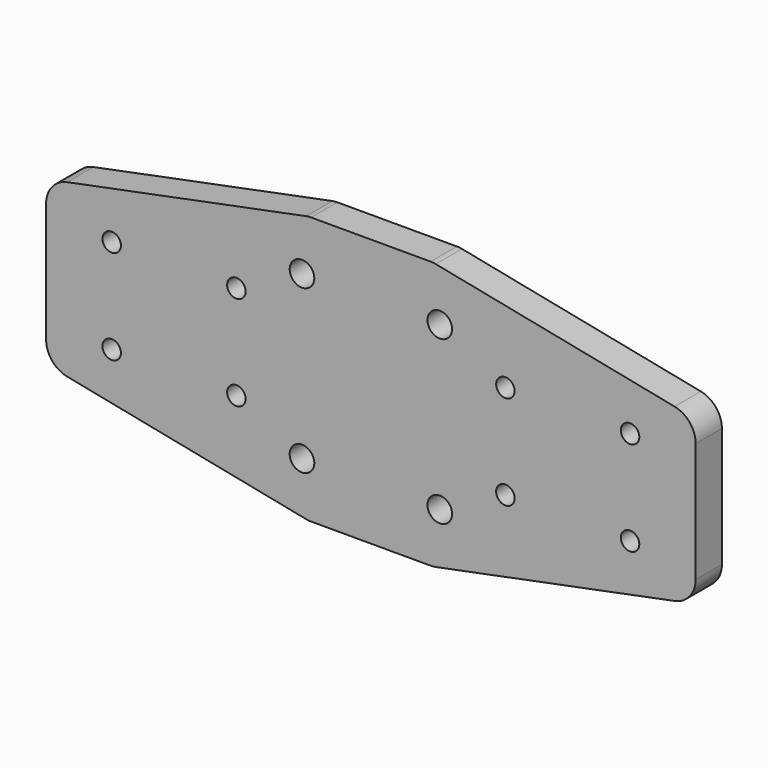
from build123d import *

# Parameters (mm, degrees)
F1_DEPTH = 6.35
F2_D     = 4.7625
F3_D     = 3.571875
F4_R     = 5.08


with BuildPart() as f1:
    # F0 (on Front) → F1 (new body)
    with BuildSketch(Plane.XZ):
        Polygon((62.865, 15.748), (12.065, 25.908), (-12.065, 25.908), (-62.865, 15.748), (-62.865, -15.748), (-12.065, -25.908), (12.065, -25.908), (62.865, -15.748), align=None)
    extrude(amount=F1_DEPTH)

    # F2 (through all)
    with Locations(Plane(origin=(0, 0, 0), x_dir=(1, 0, 0), z_dir=(0, 1, 0))):
        with Locations((-13.335, -15.748), (13.335, -15.748), (13.335, 15.748), (-13.335, 15.748)):
            Hole(F2_D / 2)

    # F3 (through all)
    with Locations(Plane(origin=(0, 0, 0), x_dir=(1, 0, 0), z_dir=(0, 1, 0))):
        with Locations((26.035, -9.144), (50.165, -9.144), (50.165, 9.144), (26.035, 9.144), (-26.035, 9.144), (-26.035, -9.144), (-50.165, -9.144), (-50.165, 9.144)):
            Hole(F3_D / 2)

    # F4
    f4_edges = [f1.edges().sort_by_distance(p)[0] for p in [
        (-62.865, -3.175, 15.748),
        (62.865, -3.175, -15.748),
        (-62.865, -3.175, -15.748),
        (62.865, -3.175, 15.748),
        (12.065, -3.175, -25.908),
        (12.065, -3.175, 25.908),
        (-12.065, -3.175, -25.908),
        (-12.065, -3.175, 25.908),
    ]]
    fillet(f4_edges, radius=F4_R)


solid = f1.part
